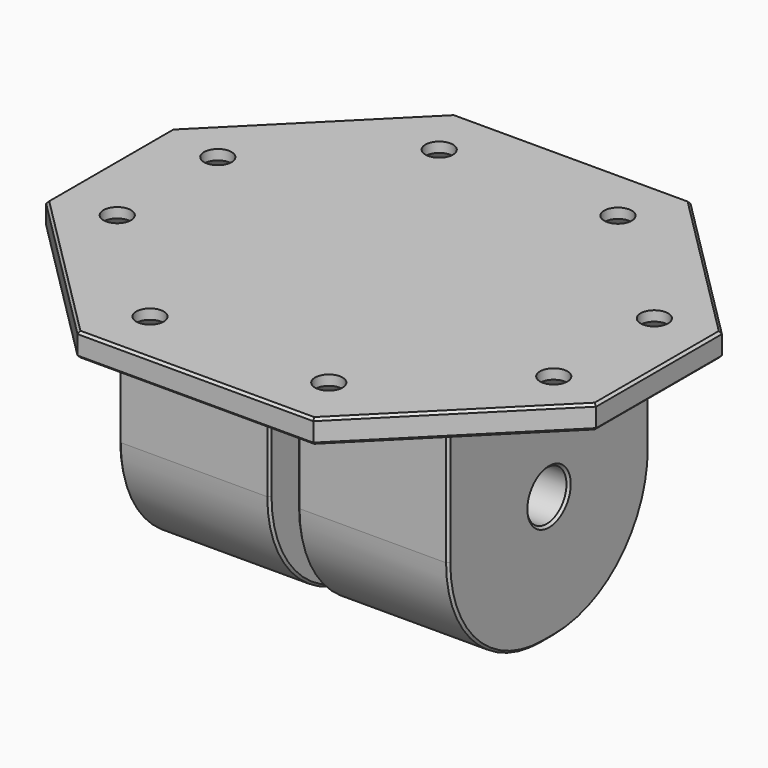
from build123d import *

# Parameters (mm, degrees)
F0_W           = 70
F0_H           = 60
F0_W_2         = 19.25
F0_H_2         = 32
F1_DEPTH       = 3
F2_DEPTH       = 32
F4_D           = 6.3
F5_R           = 15
F6_SIZE        = 20
F7_D           = 3.5
F7_CSINK_D     = 6.5
F7_CSINK_ANGLE = 82
F8_SIZE        = 0.3


# Not quite as in the source:
# - a feature names something its author has since deleted; it is built from what else it names


with BuildPart() as f1:
    # F0 (on Top) → F1 (new body)
    with BuildSketch(Plane.XY):
        Rectangle(F0_W, F0_H)
        with Locations((-11.375, 0)):
            Rectangle(F0_W_2, F0_H_2, mode=Mode.SUBTRACT)
        with Locations((11.375, 0)):
            Rectangle(F0_W_2, F0_H_2, mode=Mode.SUBTRACT)
        with Locations((11.375, 0)):
            Rectangle(F0_W_2, F0_H_2)
        with Locations((-11.375, 0)):
            Rectangle(F0_W_2, F0_H_2)
    extrude(amount=F1_DEPTH)

    # F0 (on Top) → F2 (join)
    with BuildSketch(Plane.XY):
        with Locations((-11.375, 0)):
            Rectangle(F0_W_2, F0_H_2)
        with Locations((11.375, 0)):
            Rectangle(F0_W_2, F0_H_2)
    extrude(amount=-F2_DEPTH)

    # F4 (through all)
    with Locations(Plane.YZ.offset(21)):
        with Locations((0, -16)):
            Hole(F4_D / 2)

    # F5
    f5_edges = [f1.edges().sort_by_distance(p)[0] for p in [
        (11.375, 16, -32),
        (11.375, -16, -32),
        (-11.375, -16, -32),
        (-11.375, 16, -32),
    ]]
    fillet(f5_edges, radius=F5_R)

    # F6
    f6_edges = [f1.edges().sort_by_distance(p)[0] for p in [
        (-35, 30, 1.5),
        (-35, -30, 1.5),
        (35, -30, 1.5),
        (35, 30, 1.5),
    ]]
    chamfer(f6_edges, length=F6_SIZE)

    # F7 (through all)
    with Locations(Plane(origin=(0, 0, 0), x_dir=(1, 0, 0), z_dir=(0, 0, -1))):
        with Locations((-11.375, -23), (11.375, -23), (28, -8), (28, 8), (11.375, 23), (-11.375, 23), (-27.5449063629, 8), (-27.5449063629, -8)):
            CounterSinkHole(F7_D / 2, F7_CSINK_D / 2, counter_sink_angle=F7_CSINK_ANGLE)

    # F8
    f8_edges = [f1.edges().sort_by_distance(p)[0] for p in [
        (1.75, -16, -8.5),
        (21, -16, -8.5),
        (0, -30, 0),
        (35, 0, 0),
        (0, -30, 3),
        (35, 0, 3),
        (0, 30, 3),
        (0, 30, 0),
        (-35, 0, 3),
        (-35, 0, 0),
        (-25, -20, 0),
        (-25, -20, 3),
        (-25, 20, 0),
        (-25, 20, 3),
        (25, 20, 3),
        (25, 20, 0),
        (25, -20, 3),
        (25, -20, 0),
        (-21, 16, -8.5),
        (-21, 11.606602, -27.606602),
        (-21, 0, -32),
        (-21, -16, -8.5),
        (-21, -11.606602, -27.606602),
        (-21, -3.15, -16),
        (-1.75, 16, -8.5),
        (-1.75, -16, -8.5),
        (-1.75, -11.606602, -27.606602),
        (-1.75, 0, -32),
        (-1.75, 11.606602, -27.606602),
        (-1.75, -3.15, -16),
        (1.75, 16, -8.5),
        (1.75, 11.606602, -27.606602),
        (1.75, 0, -32),
        (1.75, -11.606602, -27.606602),
        (1.75, -3.15, -16),
        (21, -11.606602, -27.606602),
        (21, 0, -32),
        (21, 16, -8.5),
        (21, 11.606602, -27.606602),
        (21, -3.15, -16),
    ]]
    chamfer(f8_edges, length=F8_SIZE)


solid = f1.part
